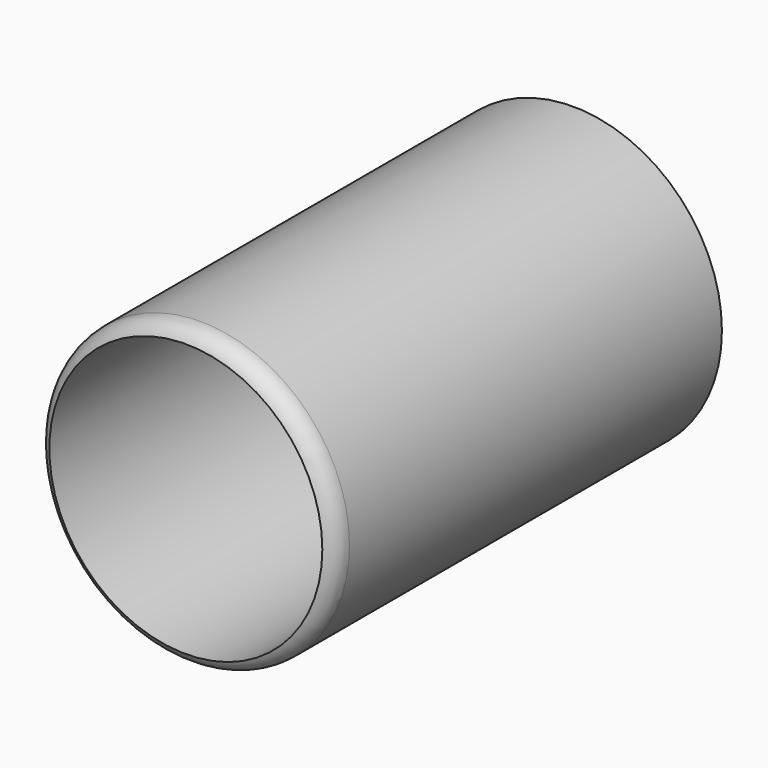
from build123d import *

# Parameters (mm, degrees)
F0_R     = 38.1
F0_R_2   = 34.925
F1_DEPTH = 123.825
F2_R     = 34.925
F3_DEPTH = 9.525


# Not quite as in the source:
# - a fillet or chamfer that OpenCascade refuses, or shapes differently, is made with other operations: its cross-section is extruded or revolved along the edge and cut away or added


with BuildPart() as f1:
    # F0 (on Front) → F1 (new body)
    with BuildSketch(Plane.XZ):
        Circle(F0_R)
        Circle(F0_R_2, mode=Mode.SUBTRACT)
    extrude(amount=F1_DEPTH)

    # F2 (on Front) → F3 (join)
    with BuildSketch(Plane.XZ):
        Circle(F2_R)
    extrude(amount=F3_DEPTH)

    # F4: fillet of radius 5.08 on 1 edges, made by hand

    # F4_s1 → F4_t2 (revolve, cut)
    with BuildSketch(Plane.XY):
        with BuildLine():
            ThreePointArc((38.1, -119.1157139607), (37.2321134838, -121.9555202921), (34.925, -123.825))
            Line((34.925, -123.825), (38.1, -123.825))
            Line((38.1, -123.825), (38.1, -119.1157139607))
        make_face()
    revolve(axis=Axis((0, -123.825, 0), (0, -1, 0)), mode=Mode.SUBTRACT)


solid = f1.part
